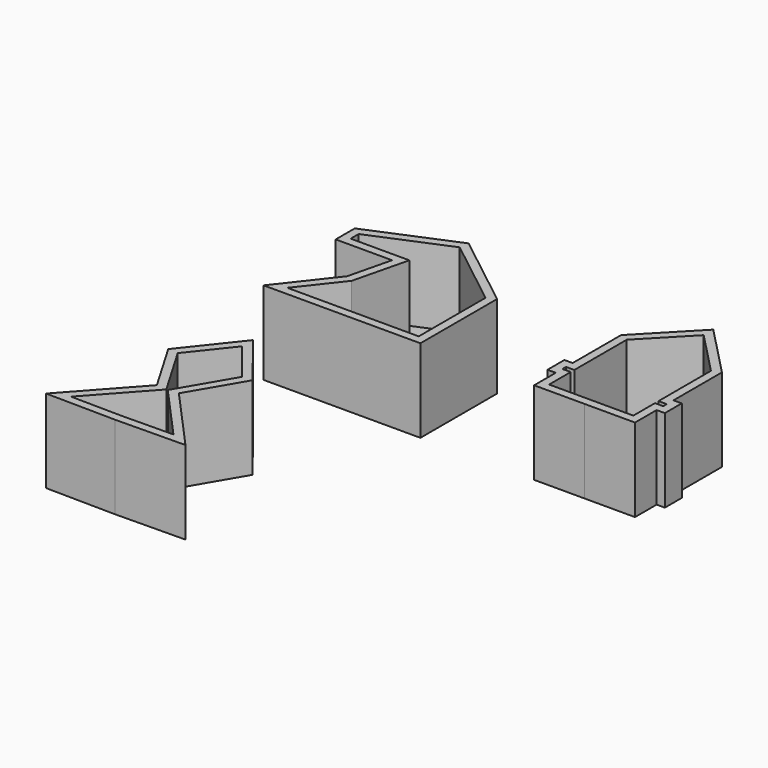
from build123d import *

# Parameters (mm, degrees)
F1_DEPTH = 25.4
F2_T     = -2.54
F4_DEPTH = 25.4
F5_T     = -2.54
F7_DEPTH = 25.4
F8_T     = -2.54


with BuildPart() as f1:
    # F0 (on Top) → F1 (new body)
    with BuildSketch(Plane.XY):
        Polygon((-44.9007153511, 16.0859264433), (-57.4897043407, 0), (-9.6515547484, 0), (-9.6515547484, 29.2344223708), (-32.8712426126, 47.418512404), (-58.8884800673, 36.5080609918), (-58.8884800673, 29.2344223708), (-41.6806784491, 29.2344223708), align=None)
    extrude(amount=F1_DEPTH)

    # F2
    f2_openings = [f1.faces().sort_by_distance(p)[0] for p in [
        (-31.482072, 20.842376, 25.4),
    ]]
    offset(amount=F2_T, openings=f2_openings, kind=Kind.INTERSECTION)


with BuildPart() as f4:
    # F3 (on Top) → F4 (new body)
    with BuildSketch(Plane.XY):
        Polygon((40.4246318837, 0), (55.8111704638, 0), (55.8111704638, 8.2527799532), (58.3289637913, 8.2527799532), (58.3289637913, 14.6871507168), (55.8111704638, 14.6871507168), (55.8111704638, 33.1509970129), (40.4246337463, 49.0970462561), (25.0380958438, 33.1509981803), (25.0380944429, 14.6871518843), (22.5203011153, 14.6871520753), (22.5203006271, 8.2527813117), (25.0380939547, 8.2527811207), (25.0380933285, 1.1675e-06), align=None)
    extrude(amount=F4_DEPTH)

    # F5
    f5_openings = [f4.faces().sort_by_distance(p)[0] for p in [
        (40.424633, 20.586239, 25.4),
    ]]
    offset(amount=F5_T, openings=f5_openings, kind=Kind.INTERSECTION)


with BuildPart() as f7:
    # F6 (on Top) → F7 (new body)
    with BuildSketch(Plane.XY):
        Polygon((-41.8234094977, -23.6393176019), (-54.6921510249, -39.8651212454), (-45.1804734766, -56.0909286141), (-63.0848109722, -75.9535506368), (-41.8234094977, -76.233305037), (-20.5620080233, -75.9535506368), (-38.4663455188, -56.0909286141), (-28.9546679705, -39.8651212454), align=None)
    extrude(amount=F7_DEPTH)

    # F8
    f8_openings = [f7.faces().sort_by_distance(p)[0] for p in [
        (-41.823409, -55.141172, 25.4),
    ]]
    offset(amount=F8_T, openings=f8_openings, kind=Kind.INTERSECTION)


solid = Compound([f1.part, f4.part, f7.part])
